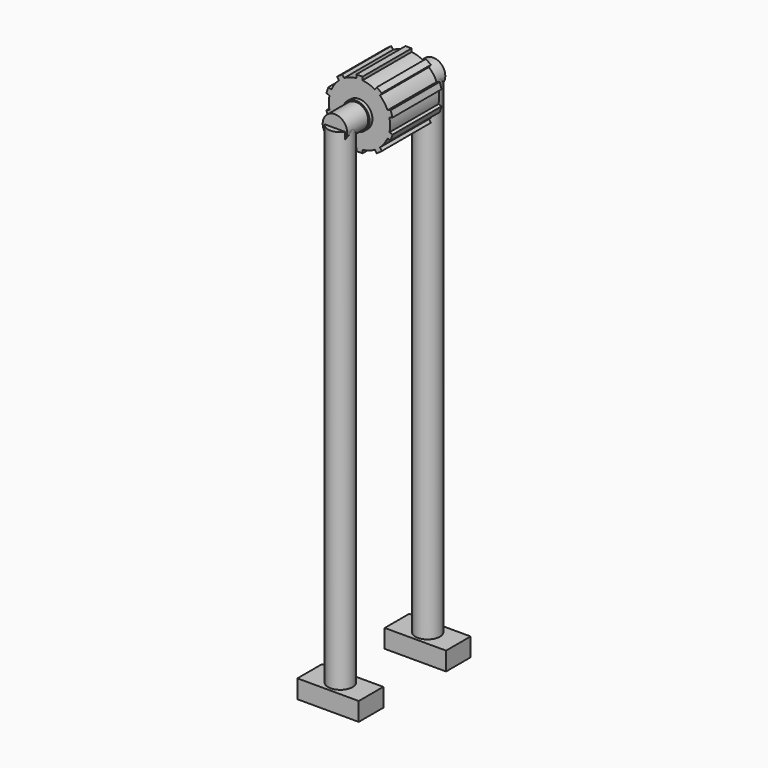
from build123d import *

# Parameters (mm, degrees)
F1_DEPTH  = 6.35
F2_R      = 2.54
F3_DEPTH  = 25.4
F4_R      = 2.5273
F5_DEPTH  = 12.7
F7_R      = 2.794
F8_DEPTH  = 0.381
F10_R     = 2.54
F11_DEPTH = 101.6
F12_W     = 12.7
F12_H     = 6.35
F13_DEPTH = 3.81


# Not quite as in the source:
# - a pattern or mirror of a feature is missing from the dataset's text; its kind, count and spacing are read off the source's solid


with BuildPart() as f1:
    # F0 (on Front) → F1 (new body, symmetric)
    with BuildSketch(Plane.XZ):
        with BuildLine():
            Line((-0.635, 6.985), (-0.635, 6.3181702256))
            ThreePointArc((-0.635, 6.3181702256), (-1.9622579143, 6.0392088785), (-3.2000014887, 5.4847507211))
            Line((-3.2000014887, 5.4847507211), (-3.5919541958, 6.0242273409))
            Line((-3.5919541958, 6.0242273409), (-4.6194057787, 5.2777400705))
            Line((-4.6194057787, 5.2777400705), (-4.2274530715, 4.7382634507))
            ThreePointArc((-4.2274530715, 4.7382634507), (-5.1372579143, 3.7324363521), (-5.8127111727, 2.5563428609))
            Line((-5.8127111727, 2.5563428609), (-6.4469039749, 2.7624045936))
            Line((-6.4469039749, 2.7624045936), (-6.8393555577, 1.5545628179))
            Line((-6.8393555577, 1.5545628179), (-6.2051627556, 1.3485010852))
            ThreePointArc((-6.2051627556, 1.3485010852), (-6.35, 0), (-6.2051627556, -1.3485010852))
            Line((-6.2051627556, -1.3485010852), (-6.8393555577, -1.5545628179))
            Line((-6.8393555577, -1.5545628179), (-6.4469039749, -2.7624045936))
            Line((-6.4469039749, -2.7624045936), (-5.8127111727, -2.5563428609))
            ThreePointArc((-5.8127111727, -2.5563428609), (-5.1372579143, -3.7324363521), (-4.2274530715, -4.7382634507))
            Line((-4.2274530715, -4.7382634507), (-4.6194057787, -5.2777400705))
            Line((-4.6194057787, -5.2777400705), (-3.5919541958, -6.0242273409))
            Line((-3.5919541958, -6.0242273409), (-3.2000014887, -5.4847507211))
            ThreePointArc((-3.2000014887, -5.4847507211), (-1.9622579143, -6.0392088785), (-0.635, -6.3181702256))
            Line((-0.635, -6.3181702256), (-0.635, -6.985))
            Line((-0.635, -6.985), (0.635, -6.985))
            Line((0.635, -6.985), (0.635, -6.3181702256))
            ThreePointArc((0.635, -6.3181702256), (1.9622579143, -6.0392088785), (3.2000014887, -5.4847507211))
            Line((3.2000014887, -5.4847507211), (3.5919541958, -6.0242273409))
            Line((3.5919541958, -6.0242273409), (4.6194057787, -5.2777400705))
            Line((4.6194057787, -5.2777400705), (4.2274530715, -4.7382634507))
            ThreePointArc((4.2274530715, -4.7382634507), (5.1372579143, -3.7324363521), (5.8127111727, -2.5563428609))
            Line((5.8127111727, -2.5563428609), (6.4469039749, -2.7624045936))
            Line((6.4469039749, -2.7624045936), (6.8393555577, -1.5545628179))
            Line((6.8393555577, -1.5545628179), (6.2051627556, -1.3485010852))
            ThreePointArc((6.2051627556, -1.3485010852), (6.35, 0), (6.2051627556, 1.3485010852))
            Line((6.2051627556, 1.3485010852), (6.8393555577, 1.5545628179))
            Line((6.8393555577, 1.5545628179), (6.4469039749, 2.7624045936))
            Line((6.4469039749, 2.7624045936), (5.8127111727, 2.5563428609))
            ThreePointArc((5.8127111727, 2.5563428609), (5.1372579143, 3.7324363521), (4.2274530715, 4.7382634507))
            Line((4.2274530715, 4.7382634507), (4.6194057787, 5.2777400705))
            Line((4.6194057787, 5.2777400705), (3.5919541958, 6.0242273409))
            Line((3.5919541958, 6.0242273409), (3.2000014887, 5.4847507211))
            ThreePointArc((3.2000014887, 5.4847507211), (1.9622579143, 6.0392088785), (0.635, 6.3181702256))
            Line((0.635, 6.3181702256), (0.635, 6.985))
            Line((0.635, 6.985), (-0.635, 6.985))
        make_face()
    extrude(amount=F1_DEPTH, both=True)

    # F2 (on face) → F3 (cut)
    with BuildSketch(Plane.XZ.offset(6.35)):
        Circle(F2_R)
    extrude(amount=-F3_DEPTH, mode=Mode.SUBTRACT)


with BuildPart() as f5:
    # F4 (on Front) → F5 (new body, symmetric)
    with BuildSketch(Plane.XZ):
        Circle(F4_R)
    extrude(amount=F5_DEPTH, both=True)

    # F7 (on offset) → F8 (join, symmetric)
    with BuildSketch(Plane.XZ.offset(6.858)):
        Circle(F7_R)
    f8 = extrude(amount=F8_DEPTH, both=True)

    # F8_copies: F8 across plane
    add(f8.mirror(Plane.ZX))

    # F10 (on offset) → F11 (join)
    with BuildSketch(Plane.XY.offset(-101.6)):
        with Locations((0, -11.2956358868)):
            Circle(F10_R)
    f11 = extrude(amount=F11_DEPTH)

    # F11_copies: F11 across plane
    add(f11.mirror(Plane(origin=(0, 0.000167, 0), x_dir=(0, 3e-06, 1), z_dir=(0, 1, -3e-06))))

    # F12 (on face) → F13 (join)
    with BuildSketch(Plane(origin=(0, 0, -101.6), x_dir=(1, 0, 0), z_dir=(0, 0, -1))):
        with Locations((0, 11.2956358868)):
            Rectangle(F12_W, F12_H)
    f13 = extrude(amount=F13_DEPTH)

    # F13_copies: F13 across plane
    add(f13.mirror(Plane.ZX))


solid = Compound([f1.part, f5.part])
